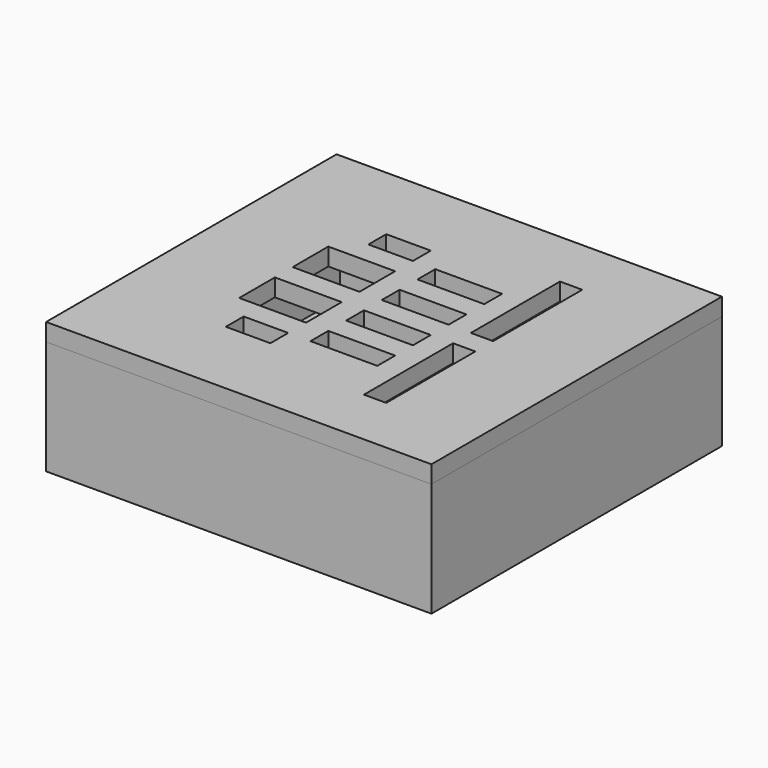
from build123d import *

# Parameters (mm, degrees)
F0_W     = 43.94
F0_H     = 41.4
F0_W_2   = 7.62
F0_H_2   = 6.95
F0_R     = 1.75
F1_DEPTH = 2
F2_DEPTH = 13
F3_DEPTH = 5
F4_W     = 43.94
F4_H     = 41.4
F4_W_2   = 5.08
F4_H_2   = 2.54
F4_W_3   = 7.62
F4_H_3   = 5.08
F4_W_4   = 2.54
F4_H_4   = 12.7
F5_DEPTH = 2


with BuildPart() as f1:
    # F0 (on Top) → F1 (new body)
    with BuildSketch(Plane.XY):
        Rectangle(F0_W, F0_H)
        Polygon((-19.97, -18.7), (-19.97, 18.7), (-5.08, 18.7), (2.54, 18.7), (19.97, 18.7), (19.97, -18.7), (2.54, -18.7), (-5.08, -18.7), align=None, mode=Mode.SUBTRACT)
        Polygon((-5.08, 18.7), (-19.97, 18.7), (-19.97, -18.7), (-5.08, -18.7), (-5.08, -11.75), (2.54, -11.75), (2.54, -18.7), (19.97, -18.7), (19.97, 18.7), (2.54, 18.7), (2.54, 11.75), (-5.08, 11.75), align=None)
        with Locations((-1.27, 15.225)):
            Rectangle(F0_W_2, F0_H_2)
        with Locations((-1.27, 15)):
            Circle(F0_R, mode=Mode.SUBTRACT)
        with Locations((-1.27, -15.225)):
            Rectangle(F0_W_2, F0_H_2)
        with Locations((-1.27, -15)):
            Circle(F0_R, mode=Mode.SUBTRACT)
    extrude(amount=F1_DEPTH)

    # F0 (on Top) → F2 (join)
    with BuildSketch(Plane.XY):
        Rectangle(F0_W, F0_H)
        Polygon((-19.97, -18.7), (-19.97, 18.7), (-5.08, 18.7), (2.54, 18.7), (19.97, 18.7), (19.97, -18.7), (2.54, -18.7), (-5.08, -18.7), align=None, mode=Mode.SUBTRACT)
    extrude(amount=F2_DEPTH)

    # F0 (on Top) → F3 (join)
    with BuildSketch(Plane.XY):
        with Locations((-1.27, 15.225)):
            Rectangle(F0_W_2, F0_H_2)
        with Locations((-1.27, 15)):
            Circle(F0_R, mode=Mode.SUBTRACT)
        with Locations((-1.27, -15.225)):
            Rectangle(F0_W_2, F0_H_2)
        with Locations((-1.27, -15)):
            Circle(F0_R, mode=Mode.SUBTRACT)
    extrude(amount=F3_DEPTH)


with BuildPart() as f5:
    # F4 (on face) → F5 (new body)
    with BuildSketch(Plane.XY.offset(13)):
        Rectangle(F4_W, F4_H)
        with Locations((-6.35, -10.16)):
            Rectangle(F4_W_2, F4_H_2, mode=Mode.SUBTRACT)
        with Locations((-7.62, -3.81)):
            Rectangle(F4_W_3, F4_H_3, mode=Mode.SUBTRACT)
        with Locations((2.54, -7.62)):
            Rectangle(F4_W_3, F4_H_2, mode=Mode.SUBTRACT)
        with Locations((10.16, -7.62)):
            Rectangle(F4_W_4, F4_H_4, mode=Mode.SUBTRACT)
        with Locations((2.54, -2.54)):
            Rectangle(F4_W_3, F4_H_2, mode=Mode.SUBTRACT)
        with Locations((-7.62, 3.81)):
            Rectangle(F4_W_3, F4_H_3, mode=Mode.SUBTRACT)
        with Locations((-6.35, 10.16)):
            Rectangle(F4_W_2, F4_H_2, mode=Mode.SUBTRACT)
        with Locations((2.54, 2.54)):
            Rectangle(F4_W_3, F4_H_2, mode=Mode.SUBTRACT)
        with Locations((2.54, 7.62)):
            Rectangle(F4_W_3, F4_H_2, mode=Mode.SUBTRACT)
        Polygon((8.89, 11.43), (8.89, 13.97), (11.43, 13.97), (11.43, 1.27), (8.89, 1.27), align=None, mode=Mode.SUBTRACT)
    extrude(amount=F5_DEPTH)


solid = Compound([f1.part, f5.part])
